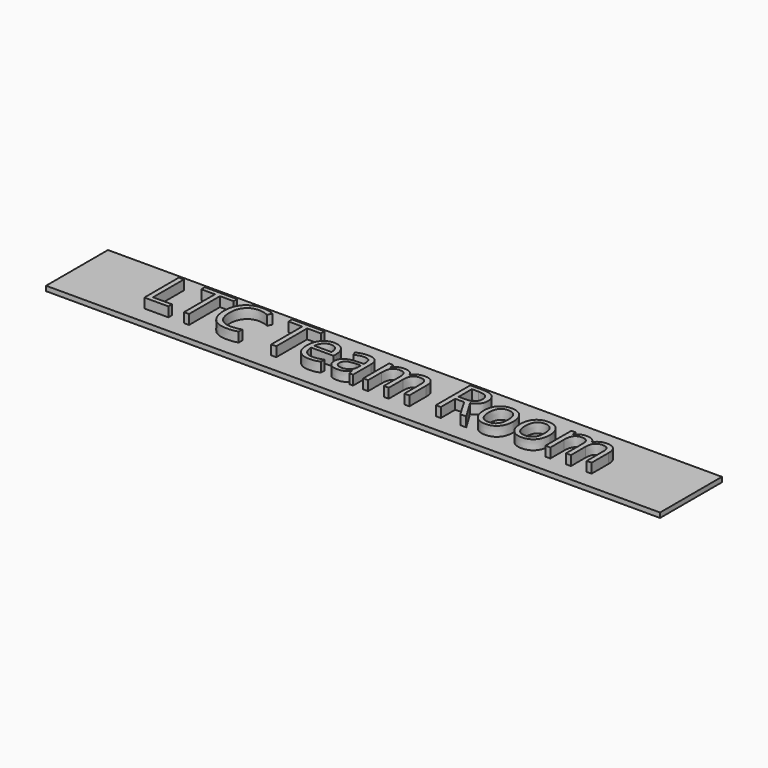
from build123d import *

# Parameters (mm, degrees)
F0_W         = 127
F0_H         = 16
F1_DEPTH     = 1
F2_TEXT_SIZE = 12.5
F3_DEPTH     = 2


# Not quite as in the source:
# - Text() gives the source's letters only with a copy of the font that has no kerning and outlines rounded to 1/6400 em; it was checked with that copy


with BuildPart() as f1:
    # F0 (on Top) → F1 (new body)
    with BuildSketch(Plane.XY):
        Rectangle(F0_W, F0_H)
    extrude(amount=F1_DEPTH)

    # F2 (on face) → F3 (join)
    with BuildSketch(Plane.XY.offset(1)):
        with Locations((-47.3509622192, -4.3087269338)):
            Text('LTC Team Room', F2_TEXT_SIZE, font='Open Sans', text_align=(TextAlign.LEFT, TextAlign.BOTTOM))
    extrude(amount=F3_DEPTH)


solid = f1.part
